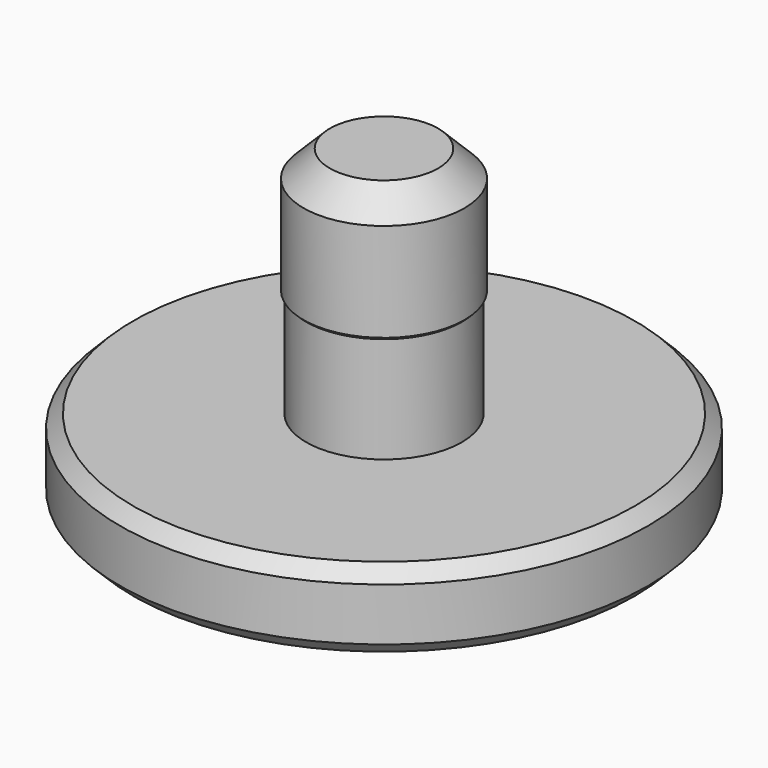
from build123d import *

# Parameters (mm, degrees)
F0_R        = 10
F1_DEPTH    = 3
F2_R        = 2.95
F3_DEPTH    = 3.61
F4_R        = 3.05
F4_R_2      = 2.95
F5_DEPTH    = 5.23
F6_SIZE     = 1
F7_SIZE     = 0.5
F8_S5_R     = 2.95
F8_T6_DEPTH = 6


# Not quite as in the source:
# - a fillet or chamfer that OpenCascade refuses, or shapes differently, is made with other operations: its cross-section is extruded or revolved along the edge and cut away or added


with BuildPart() as f1:
    # F0 (on Top) → F1 (new body)
    with BuildSketch(Plane.XY):
        Circle(F0_R)
    extrude(amount=F1_DEPTH)

    # F2 (on face) → F3 (join)
    with BuildSketch(Plane.XY.offset(3)):
        Circle(F2_R)
    extrude(amount=F3_DEPTH)

    # F4 (on face) → F5 (join)
    with BuildSketch(Plane.XY.offset(6.61)):
        Circle(F4_R)
        Circle(F4_R_2, mode=Mode.SUBTRACT)
        Circle(F4_R_2)
    extrude(amount=F5_DEPTH)

    # F6
    f6_edges = [f1.edges().sort_by_distance(p)[0] for p in [
        (-3.05, 0, 11.84),
    ]]
    chamfer(f6_edges, length=F6_SIZE)

    # F7
    f7_edges = [f1.edges().sort_by_distance(p)[0] for p in [
        (-10, 0, 3),
        (-10, 0, 0),
    ]]
    chamfer(f7_edges, length=F7_SIZE)

    # F8: chamfer of 0.5 on 1 edges, made by hand


with BuildPart() as f8_tool2:
    # F8_s3 → F8_t4 (revolve)
    with BuildSketch(Plane.XZ):
        Polygon((2.55, 6.61), (3.05, 7.11), (3.05, 6.61), align=None)
    revolve(axis=Axis((0, 0, 6.61), (0, 0, 1)))

    # F8_s5 → F8_t6 (cut, symmetric)
    with BuildSketch(Plane.XY.offset(6.9)):
        Circle(F8_S5_R)
    extrude(amount=F8_T6_DEPTH, both=True, mode=Mode.SUBTRACT)


with BuildPart() as f1_1:
    add(f1.part)

    # F8_t1: cut F8_tool2
    add(f8_tool2.part, mode=Mode.SUBTRACT)


solid = f1_1.part
